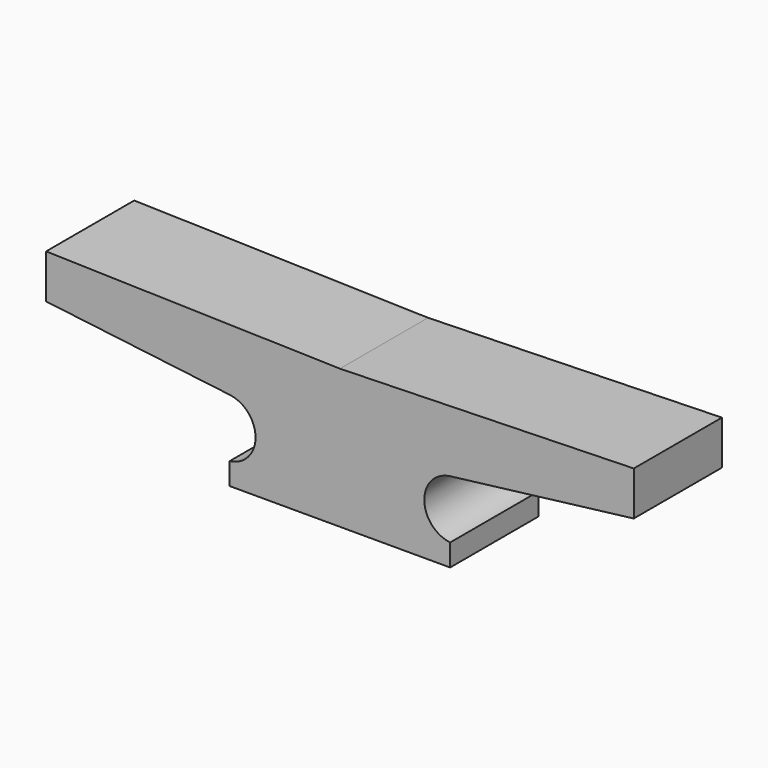
from build123d import *

# Parameters (mm, degrees)
F2_DEPTH = 19.05


# Not quite as in the source:
# - a variable given as a bare number and used for a length is read in inches; the dataset says mm whatever the document's units were


with BuildPart() as f2:
    # F1 (on Front) → F2 (new body)
    with BuildSketch(Plane.XZ):
        with BuildLine():
            Line((0, 24.0697551843), (-50.8, 25.4))
            Line((-50.8, 25.4), (-50.8, 17.78))
            Line((-50.8, 17.78), (-19.05, 13.8947746143))
            ThreePointArc((-19.05, 13.8947746143), (-14.5870334227, 8.8523873071), (-19.05, 3.81))
            Line((-19.05, 3.81), (-19.05, 0))
            Line((-19.05, 0), (0, 0))
            Line((0, 0), (19.05, 0))
            Line((19.05, 0), (19.05, 3.81))
            ThreePointArc((19.05, 3.81), (14.5870334227, 8.8523873071), (19.05, 13.8947746143))
            Line((19.05, 13.8947746143), (50.8, 17.78))
            Line((50.8, 17.78), (50.8, 25.4))
            Line((50.8, 25.4), (0, 24.0697551843))
        make_face()
    extrude(amount=F2_DEPTH)


solid = f2.part
